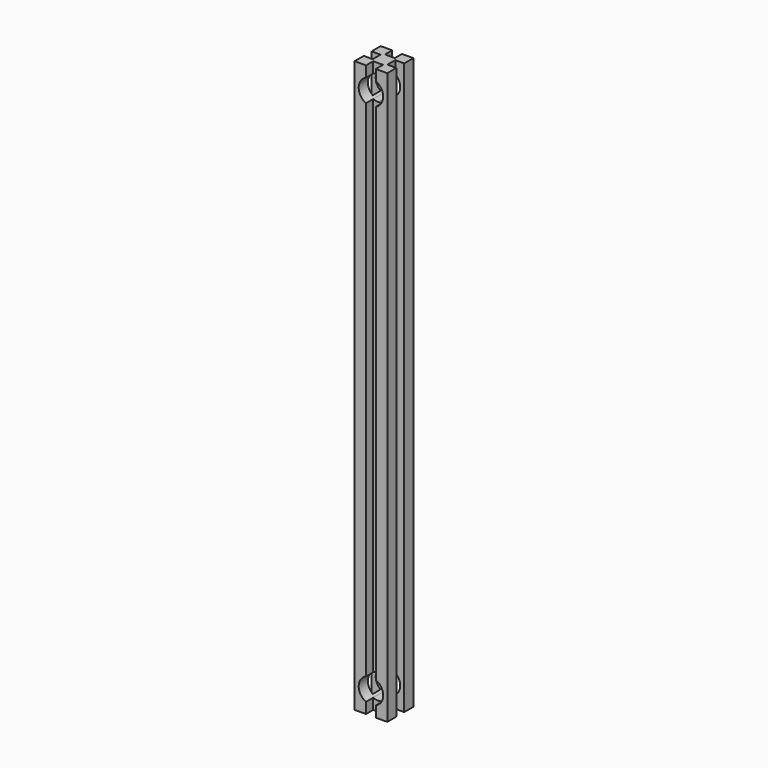
from build123d import *

# Parameters (mm, degrees)
F1_DEPTH = 350
F3_DEPTH = 25


with BuildPart() as f1:
    # F0 (on Top) → F1 (new body)
    with BuildSketch(Plane.XY):
        Polygon((0, 7), (0, 0), (7, 0), (7, 5.5), (13, 5.5), (13, 0), (20, 0), (20, 7), (14.5, 7), (14.5, 13), (20, 13), (20, 20), (13, 20), (13, 14.5), (7, 14.5), (7, 20), (0, 20), (0, 13), (5.5, 13), (5.5, 7), align=None)
    extrude(amount=F1_DEPTH)

    # F2 (on face) → F3 (cut)
    with BuildSketch(Plane.XZ):
        with BuildLine():
            ThreePointArc((7, 329.6261364576), (8.4676776723, 329.158202653), (10, 329))
            ThreePointArc((10, 329), (15.3033008589, 331.1966991411), (17.5, 336.5))
            ThreePointArc((17.5, 336.5), (14.1079191813, 342.774950199), (7, 343.3738635424))
            Line((7, 343.3738635424), (7, 329.6261364576))
        make_face()
        with BuildLine():
            ThreePointArc((7, 343.3738635424), (2.5, 336.5), (7, 329.6261364576))
            Line((7, 329.6261364576), (7, 343.3738635424))
        make_face()
        with BuildLine():
            Line((7, 6.6261364576), (7, 20.3738635424))
            ThreePointArc((7, 20.3738635424), (2.5, 13.5), (7, 6.6261364576))
        make_face()
        with BuildLine():
            ThreePointArc((10, 21), (8.4676776723, 20.841797347), (7, 20.3738635424))
            Line((7, 20.3738635424), (7, 6.6261364576))
            ThreePointArc((7, 6.6261364576), (14.1079191813, 7.225049801), (17.5, 13.5))
            ThreePointArc((17.5, 13.5), (15.3033008589, 18.8033008589), (10, 21))
        make_face()
    extrude(amount=-F3_DEPTH, mode=Mode.SUBTRACT)


solid = f1.part
